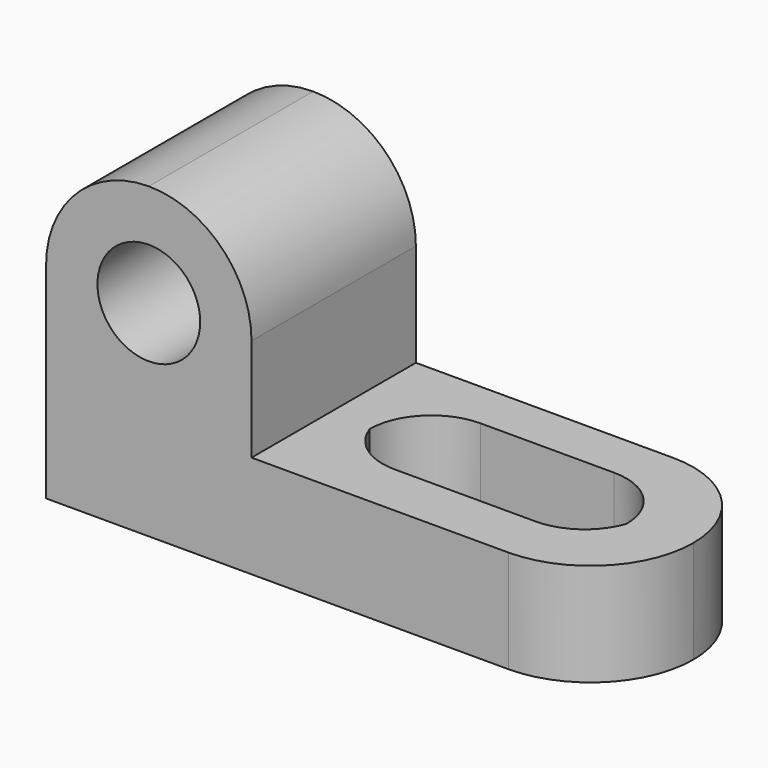
from build123d import *

# Parameters (mm, degrees)
F1_DEPTH     = 25.4
F2_R         = 12.7
F3_R         = 12.69999
F4_R         = 12.7
F5_R         = 12.69999
F6_R         = 6.35
F7_DEPTH     = 25.4
F8_W         = 31.75
F8_H         = 12.7
F9_DEPTH     = 25.4
F10_R        = 7.62
F11_T1_DEPTH = 12.7
F12_R        = 7.62
F13_T1_DEPTH = 12.7


# Not quite as in the source:
# - a fillet or chamfer that OpenCascade refuses, or shapes differently, is made with other operations: its cross-section is extruded or revolved along the edge and cut away or added
# - a fillet or chamfer is up to 0.001 mm smaller than in the source, because OpenCascade refuses the exact size


with BuildPart() as f1:
    # F0 (on Front) → F1 (new body)
    with BuildSketch(Plane.XZ):
        Polygon((0, 38.1), (0, 0), (69.85, 0), (69.85, 12.7), (25.4, 12.7), (25.4, 38.1), align=None)
    extrude(amount=F1_DEPTH)

    # F2
    f2_edges = [f1.edges().sort_by_distance(p)[0] for p in [
        (69.85, -25.4, 6.35),
    ]]
    fillet(f2_edges, radius=F2_R)

    # F3 (radius 12.7 in the source; OpenCascade refuses exactly that, so slightly less here)
    f3_edges = [f1.edges().sort_by_distance(p)[0] for p in [
        (69.85, 0, 6.35),
    ]]
    fillet(f3_edges, radius=F3_R)

    # F4
    f4_edges = [f1.edges().sort_by_distance(p)[0] for p in [
        (25.4, -12.7, 38.1),
    ]]
    fillet(f4_edges, radius=F4_R)

    # F5 (radius 12.7 in the source; OpenCascade refuses exactly that, so slightly less here)
    f5_edges = [f1.edges().sort_by_distance(p)[0] for p in [
        (0, -12.7, 38.1),
    ]]
    fillet(f5_edges, radius=F5_R)

    # F6 (on face) → F7 (cut)
    with BuildSketch(Plane.XZ.offset(25.4)):
        with Locations((12.7, 25.4)):
            Circle(F6_R)
    extrude(amount=-F7_DEPTH, mode=Mode.SUBTRACT)

    # F8 (on face) → F9 (cut)
    with BuildSketch(Plane.XY.offset(12.7)):
        with Locations((46.4384327233, -12.3384663999)):
            Rectangle(F8_W, F8_H)
    extrude(amount=-F9_DEPTH, mode=Mode.SUBTRACT)

    # F10
    f10_edges = [f1.edges().sort_by_distance(p)[0] for p in [
        (30.563433, -5.988466, 6.35),
    ]]
    fillet(f10_edges, radius=F10_R)

    # F11: fillet of radius 7.62 on 1 edges, made by hand

    # F11_s2 → F11_t1 (join)
    with BuildSketch(Plane.XY):
        with BuildLine():
            ThreePointArc((30.5634327233, -13.6084663999), (33.3482285689, -17.2901703466), (37.7476376201, -18.6884663999))
            Line((37.7476376201, -18.6884663999), (30.5634327233, -18.6884663999))
            Line((30.5634327233, -18.6884663999), (30.5634327233, -13.6084663999))
        make_face()
    extrude(amount=F11_T1_DEPTH)

    # F12
    f12_edges = [f1.edges().sort_by_distance(p)[0] for p in [
        (62.313433, -5.988466, 6.35),
    ]]
    fillet(f12_edges, radius=F12_R)

    # F13: fillet of radius 7.62 on 1 edges, made by hand

    # F13_s2 → F13_t1 (join)
    with BuildSketch(Plane.XY):
        with BuildLine():
            ThreePointArc((62.3134327233, -13.6084663999), (59.5286368777, -17.2901703466), (55.1292278264, -18.6884663999))
            Line((55.1292278264, -18.6884663999), (62.3134327233, -18.6884663999))
            Line((62.3134327233, -18.6884663999), (62.3134327233, -13.6084663999))
        make_face()
    extrude(amount=F13_T1_DEPTH)


solid = f1.part
